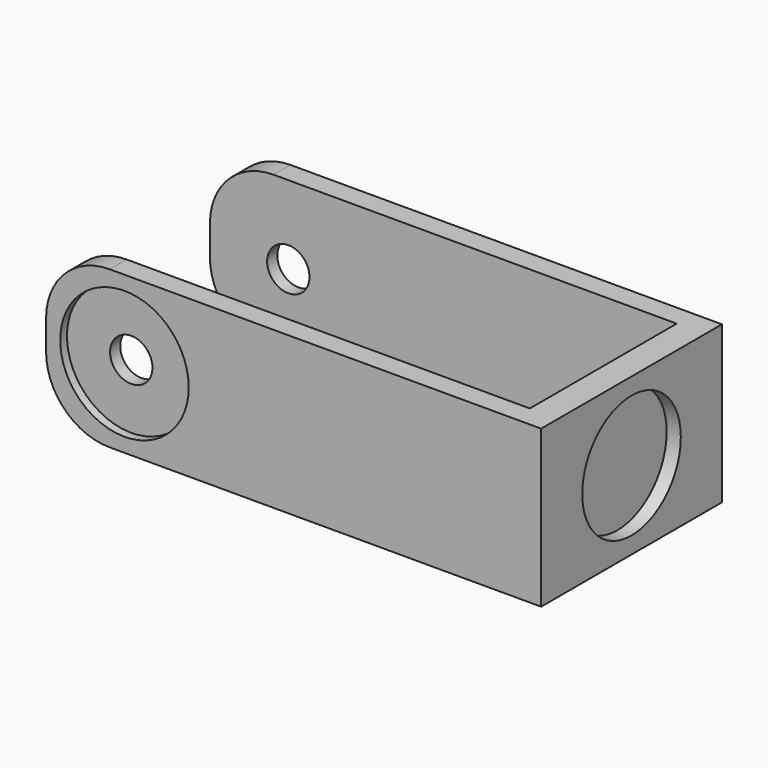
from build123d import *

# Parameters (mm, degrees)
F0_R     = 9.1
F0_R_2   = 3
F1_DEPTH = 3
F0_W     = 25
F0_H     = 4
F2_DEPTH = 32
F3_R     = 9.1
F3_R_2   = 3
F4_DEPTH = 3
F5_DEPTH = 1.2
F6_R     = 8.725
F7_DEPTH = 2
F8_DEPTH = 1.2


# Not quite as in the source:
# - a feature names something its author has since deleted; it is built from what else it names


with BuildPart() as f1:
    # F0 (on Front) → F1 (new body)
    with BuildSketch(Plane.XZ):
        with BuildLine():
            Line((55, 11.1), (-2.1, 11.1))
            ThreePointArc((-2.1, 11.1), (-8.4639610307, 8.4639610307), (-11.1, 2.1))
            Line((-11.1, 2.1), (-11.1, -2.1))
            ThreePointArc((-11.1, -2.1), (-8.4639610307, -8.4639610307), (-2.1, -11.1))
            Line((-2.1, -11.1), (30, -11.1))
            Line((30, -11.1), (30, -7.1))
            Line((30, -7.1), (55, -7.1))
            Line((55, -7.1), (55, 11.1))
        make_face()
        Circle(F0_R, mode=Mode.SUBTRACT)
        Circle(F0_R)
        Circle(F0_R_2, mode=Mode.SUBTRACT)
    extrude(amount=-F1_DEPTH)

    # F0 (on Front) → F2 (join)
    with BuildSketch(Plane.XZ):
        Polygon((59, 11.1), (55, 11.1), (55, -7.1), (55, -11.1), (59, -11.1), align=None)
        with Locations((42.5, -9.1)):
            Rectangle(F0_W, F0_H)
    extrude(amount=-F2_DEPTH)

    # F3 (on face) → F4 (join)
    with BuildSketch(Plane(origin=(0, 32, 0), x_dir=(-1, 0, 0), z_dir=(0, 1, 0))):
        with BuildLine():
            Line((-30, -7.1), (-30, -11.1))
            Line((-30, -11.1), (2.1, -11.1))
            ThreePointArc((2.1, -11.1), (8.4639610307, -8.4639610307), (11.1, -2.1))
            Line((11.1, -2.1), (11.1, 2.1))
            ThreePointArc((11.1, 2.1), (8.4639610307, 8.4639610307), (2.1, 11.1))
            Line((2.1, 11.1), (-55, 11.1))
            Line((-55, 11.1), (-55, -7.1))
            Line((-55, -7.1), (-30, -7.1))
        make_face()
        Circle(F3_R, mode=Mode.SUBTRACT)
        Circle(F3_R)
        Circle(F3_R_2, mode=Mode.SUBTRACT)
    extrude(amount=-F4_DEPTH)

    # F0 (on Front) → F5 (cut)
    with BuildSketch(Plane.XZ):
        Circle(F0_R)
        Circle(F0_R_2, mode=Mode.SUBTRACT)
    extrude(amount=-F5_DEPTH, mode=Mode.SUBTRACT)

    # F6 (on face) → F7 (cut)
    with BuildSketch(Plane.YZ.offset(59)):
        with Locations((16, 0)):
            Circle(F6_R)
    extrude(amount=-F7_DEPTH, mode=Mode.SUBTRACT)

    # F3 (on face) → F8 (cut)
    with BuildSketch(Plane(origin=(0, 32, 0), x_dir=(-1, 0, 0), z_dir=(0, 1, 0))):
        Circle(F3_R)
        Circle(F3_R_2, mode=Mode.SUBTRACT)
    extrude(amount=-F8_DEPTH, mode=Mode.SUBTRACT)


solid = f1.part
